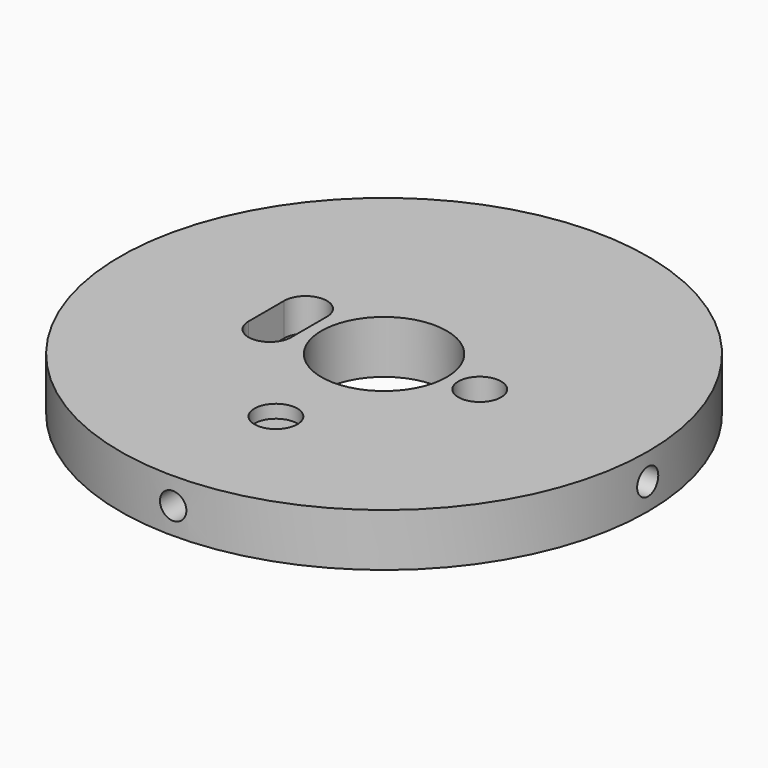
from build123d import *

# Parameters (mm, degrees)
F0_R             = 40
F1_DEPTH         = 8
F2_R             = 9.5
F3_DEPTH         = 8.001
F5_R             = 3.25
F6_DEPTH         = 4
F8_DEPTH         = 5
F9_R             = 3.25
F10_DEPTH        = 2
F12_R            = 2
F13_DEPTH        = 15
F13_COPIES_COUNT = 4


# Not quite as in the source:
# - a pattern or mirror of a feature is missing from the dataset's text; its kind, count and spacing are read off the source's solid


with BuildPart() as f1:
    # F0 (on Top) → F1 (new body)
    with BuildSketch(Plane.XY):
        Circle(F0_R)
    extrude(amount=F1_DEPTH)

    # F2 (on face) → F3 (cut, through all)
    with BuildSketch(Plane.XY.offset(8)):
        Circle(F2_R)
    extrude(amount=-F3_DEPTH, mode=Mode.SUBTRACT)

    # F5 (on face) → F6 (cut)
    with BuildSketch(Plane.XY.offset(8)):
        with Locations((14.5, 0)):
            Circle(F5_R)
    extrude(amount=-F6_DEPTH, mode=Mode.SUBTRACT)

    # F7 (on face) → F8 (cut)
    with BuildSketch(Plane.XY.offset(8)):
        with BuildLine():
            Line((-17.75, 3.25), (-17.75, -3.5))
            ThreePointArc((-17.75, -3.5), (-14.5, -6.75), (-11.25, -3.5))
            Line((-11.25, -3.5), (-11.25, 3.25))
            ThreePointArc((-11.25, 3.25), (-14.5, 6.5), (-17.75, 3.25))
        make_face()
    extrude(amount=-F8_DEPTH, mode=Mode.SUBTRACT)

    # F9 (on face) → F10 (cut)
    with BuildSketch(Plane.XY.offset(8)):
        with Locations((0, -20.4880452948)):
            Circle(F9_R)
    extrude(amount=-F10_DEPTH, mode=Mode.SUBTRACT)

    # F12 (on offset) → F13 (cut)
    with BuildSketch(Plane.XZ.offset(40.792)):
        with Locations((0, 4)):
            Circle(F12_R)
    f13 = extrude(amount=-F13_DEPTH, mode=Mode.SUBTRACT)

    # F13_copies: F13 ×4 about axis
    f13_copies_axis = Axis((0, 0, 0), (0, 0, 1))
    for i in range(1, F13_COPIES_COUNT):
        add(f13.rotate(f13_copies_axis, i * 360 / F13_COPIES_COUNT), mode=Mode.SUBTRACT)


solid = f1.part
